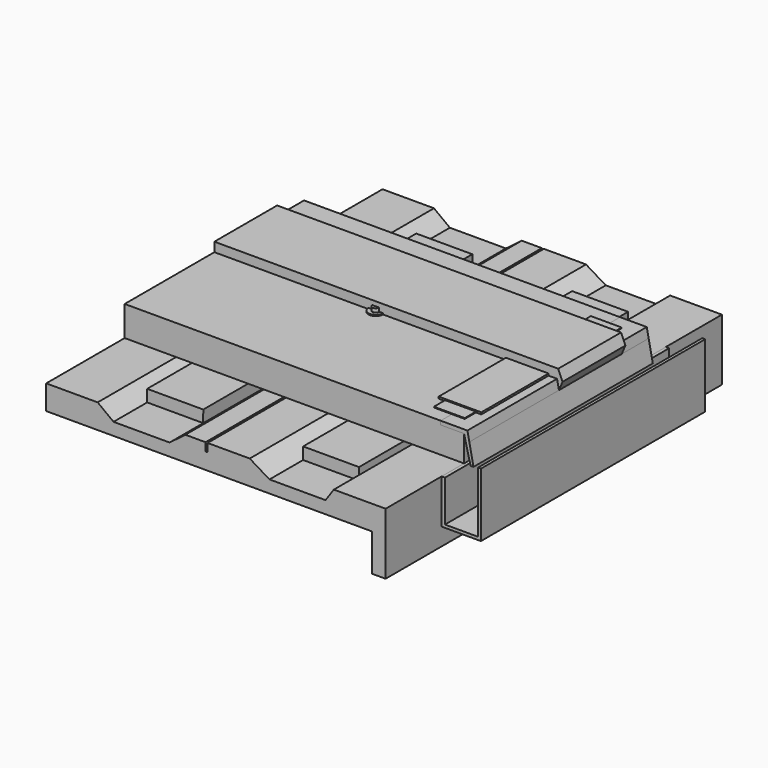
from build123d import *

# Parameters (mm, degrees)
F1_DEPTH  = 190.5
F2_DEPTH  = 152.4
F0_W      = 1.8636145309
F0_H      = 27.2141208457
F3_DEPTH  = 101.6
F0_H_2    = 3.1851885769
F0_H_3    = 7.4091651964
F6_DEPTH  = 127
F7_DEPTH  = 101.6
F8_DEPTH  = 88.9
F9_DEPTH  = 76.2
F10_DEPTH = 71.12


with BuildPart() as f1:
    # F0 (on Front) → F1 (new body, symmetric)
    with BuildSketch(Plane.XZ):
        Polygon((-127.1288654061, 3.3602740393), (-173.7859473037, 3.3602740393), (-173.8923100857, -18.7623016536), (121.4632987976, -18.7623016536), (121.4632987976, -52.5190801178), (133.8279108456, -52.5190801178), (133.8279108456, -36.7227010429), (133.8279108456, 3.3609198822), (86.8995636396, 3.3609198822), (79.3755978542, -7.4902105568), (28.5755978542, -7.4902105568), (10.6749085502, 3.3609198822), (-27.5120586157, 3.3609198822), (-27.5120586157, -4.0482453142), (-29.3756731466, -4.0482453142), (-29.3756731466, 3.3609198822), (-47.6464486061, 3.3609198822), (-61.951972467, -7.4902105568), (-112.751972467, -7.4902105568), align=None)
    extrude(amount=F1_DEPTH, both=True)


with BuildPart() as f2:
    # F0 (on Front) → F2 (new body, symmetric)
    with BuildSketch(Plane.XZ):
        Polygon((-112.751972467, 3.3609198822), (-112.751972467, -7.4902105568), (-61.951972467, -7.4902105568), (-61.9183145463, 3.3609198822), align=None)
    extrude(amount=F2_DEPTH, both=True)


with BuildPart() as f2b:
    # F0 (on Front) → F2, piece 2 (new body, symmetric)
    with BuildSketch(Plane.XZ):
        Polygon((28.5755978542, 3.3609198822), (28.5755978542, -7.4902105568), (79.3755978542, -7.4902105568), (79.2492181063, 3.3609198822), align=None)
    extrude(amount=F2_DEPTH, both=True)


with BuildPart() as f3:
    # F0 (on Front) → F3 (new body, symmetric)
    with BuildSketch(Plane.XZ):
        Polygon((90.4897078872, 30.5750407279), (-27.5120586157, 30.5750407279), (-27.5120586157, 3.3609198822), (10.6749085502, 3.3609198822), (28.5755978542, 3.3609198822), (79.2492181063, 3.3609198822), (86.8995636396, 3.3609198822), (133.8279108456, 3.3609198822), (133.8279108456, 27.1575767547), (112.6352027059, 27.1575767547), (112.6352027059, 30.5750407279), (96.3365361094, 30.5750407279), align=None)
        Polygon((-173.7859473037, 30.5750407279), (-173.7859473037, 3.3602740393), (-127.1288654061, 3.3602740393), (-112.751972467, 3.3609198822), (-61.9183145463, 3.3609198822), (-47.6464486061, 3.3609198822), (-29.3756731466, 3.3609198822), (-29.3756731466, 30.5750407279), (-34.1368317604, 30.5750407279), align=None)
        with Locations((-28.4438658811, 16.967980305)):
            Rectangle(F0_W, F0_H)
    extrude(amount=F3_DEPTH, both=True)


with BuildPart() as f4:
    # F0 (on Front) → F4 (revolve)
    with BuildSketch(Plane.XZ):
        with Locations((-28.4438658811, 32.1676350163)):
            Rectangle(F0_W, F0_H_2)
        with Locations((-28.4438658811, 16.967980305)):
            Rectangle(F0_W, F0_H)
        with Locations((-28.4438658811, -0.343662716)):
            Rectangle(F0_W, F0_H_3)
    revolve(axis=Axis((-27.5120586157, 0, 14.7883250342), (0, 0, -1)))


with BuildPart() as f5:
    # F0 (on Front) → F5 (revolve)
    with BuildSketch(Plane.XZ):
        Polygon((-34.1368317604, 31.5995030105), (-34.1368317604, 30.5750407279), (-29.3756731466, 30.5750407279), (-29.3756731466, 33.7602293047), (-27.5120586157, 33.7602293047), (-27.5120586157, 34.9623337388), (-30.6394901127, 34.9623337388), (-30.6394901127, 31.5995030105), align=None)
    revolve(axis=Axis((-27.5120586157, 0, 14.7883250342), (0, 0, -1)))


with BuildPart() as f6:
    # F0 (on Front) → F6 (new body, symmetric)
    with BuildSketch(Plane.XZ):
        Polygon((133.8279108456, 3.3609198822), (133.8279108456, -36.7227010429), (169.4176793098, -36.7227010429), (169.4176793098, 21.1112946272), (166.7888611555, 21.1112946272), (166.7888611555, -34.0938866138), (136.8203312159, -34.0938866138), (136.8203312159, 3.3609198822), align=None)
    extrude(amount=F6_DEPTH, both=True)


with BuildPart() as f7:
    # F0 (on Front) → F7 (new body, symmetric)
    with BuildSketch(Plane.XZ):
        Polygon((124.2782771587, 30.5750407279), (112.6352027059, 30.5750407279), (112.6352027059, 27.1575767547), (133.8279108456, 27.1575767547), (133.8279108456, 30.5750407279), (129.1052103043, 30.5750407279), align=None)
        Polygon((142.3408389091, 3.3602740393), (138.5535198667, 22.0308401975), (136.8203312159, 30.5750407279), (133.8279108456, 30.5750407279), (133.8279108456, 27.1575767547), (139.712035656, 3.3602740393), align=None)
    extrude(amount=F7_DEPTH, both=True)


with BuildPart() as f8:
    # F0 (on Front) → F8 (new body, symmetric)
    with BuildSketch(Plane.XZ):
        Polygon((96.3365361094, 31.289357692), (96.3365361094, 30.5750407279), (112.6352027059, 30.5750407279), (124.2782771587, 30.5750407279), (124.2782771587, 31.289357692), align=None)
    extrude(amount=F8_DEPTH, both=True)


with BuildPart() as f9:
    # F0 (on Front) → F9 (new body, symmetric)
    with BuildSketch(Plane.XZ):
        Polygon((90.4897078872, 32.3055572808), (90.4897078872, 30.5750407279), (96.3365361094, 30.5750407279), (96.3365361094, 31.289357692), (124.2782771587, 31.289357692), (124.2782771587, 30.5750407279), (129.1052103043, 30.5750407279), (129.1052103043, 32.3055572808), align=None)
    extrude(amount=F9_DEPTH, both=True)


with BuildPart() as f10:
    # F0 (on Front) → F10 (new body)
    with BuildSketch(Plane.XZ):
        Polygon((-173.7859473037, 38.9586053789), (-173.7859473037, 30.5750407279), (-34.1368317604, 30.5750407279), (-34.1368317604, 31.5995030105), (-30.6394901127, 31.5995030105), (-30.6394901127, 34.9623337388), (-27.5120586157, 34.9623337388), (-27.5120586157, 33.7602293047), (-27.5120586157, 30.5750407279), (90.4897078872, 30.5750407279), (90.4897078872, 32.3055572808), (129.1052103043, 32.3055572808), (129.1052103043, 30.5750407279), (133.8279108456, 30.5750407279), (136.8203312159, 30.5750407279), (138.5535198667, 22.0308401975), (141.8251693249, 29.8087727278), (137.8684788942, 38.9586053789), align=None)
    extrude(amount=-F10_DEPTH)


solid = Compound([f1.part, f2.part, f2b.part, f3.part, f4.part, f5.part, f6.part, f7.part, f8.part, f9.part, f10.part])
